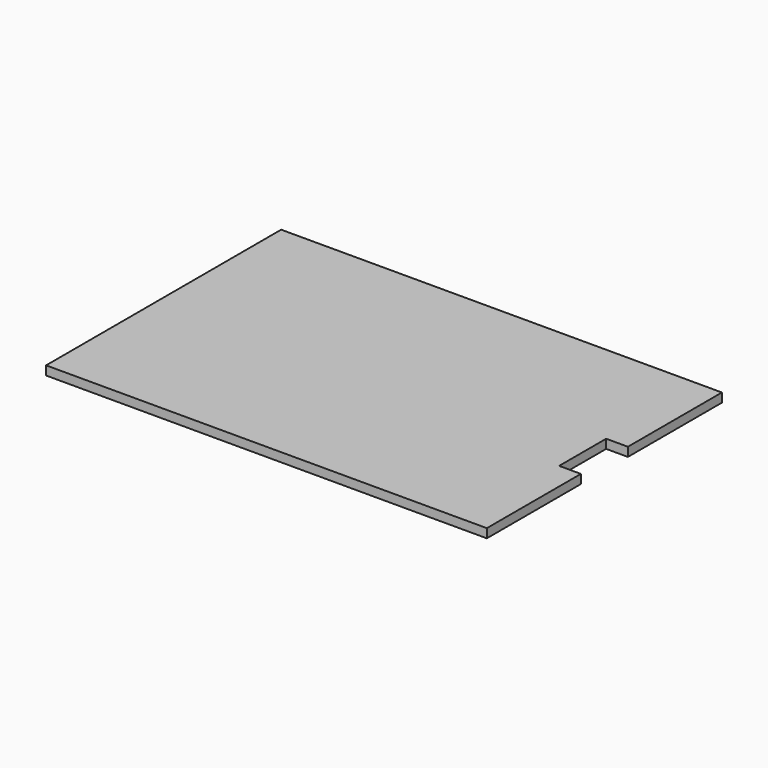
from build123d import *

# Parameters (mm, degrees)
F1_DEPTH = 3.1


# Not quite as in the source:
# - a feature names something its author has since deleted; it is built from what else it names


with BuildPart() as f1:
    # F0 (on Top) → F1 (new body)
    with BuildSketch(Plane.XY):
        Polygon((0, 101.6), (0, 0), (152.4, 0), (152.4, 40.64), (144.8868364096, 40.64), (144.8868364096, 60.96), (152.4, 60.96), (152.4, 101.6), align=None)
    extrude(amount=F1_DEPTH)


solid = f1.part
